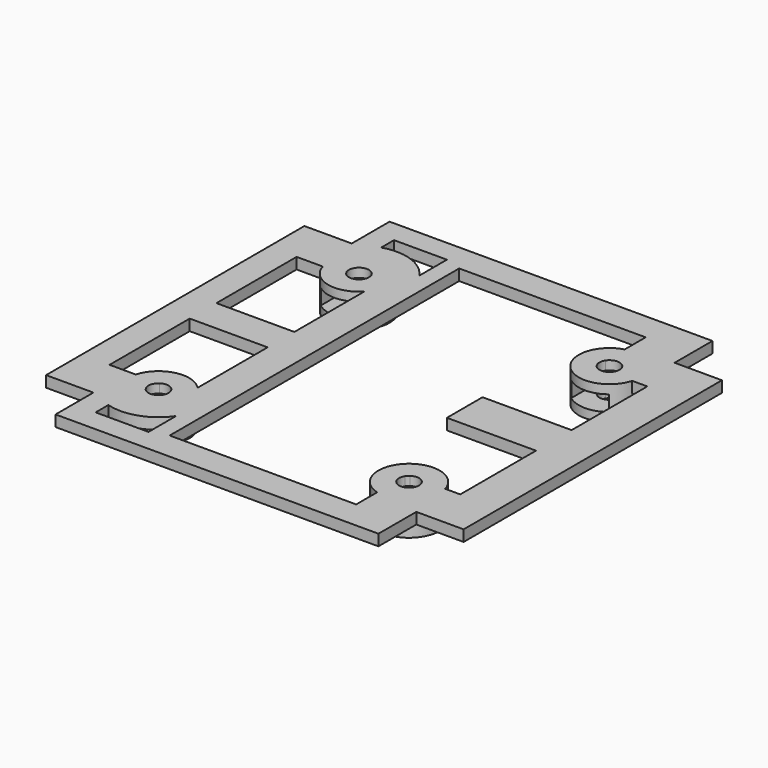
from build123d import *

# Parameters (mm, degrees)
F2_DEPTH       = 2
F3_W           = 13.9999988079
F3_H           = 18
F4_DEPTH       = 2.001
F6_DEPTH       = 6
F7_R           = 1.8
F8_DEPTH       = 6.001
F10_R          = 3.4
F11_DEPTH      = 1.4
F11_DEPTH_BACK = 1.4
F13_W          = 6.8
F13_H          = 2.8
F14_DEPTH      = 8.8
F16_W          = 6.8
F16_H          = 2.8
F17_DEPTH      = 10.3
F18_W          = 8
F18_H          = 2
F19_DEPTH      = 16
F21_DEPTH      = 2.001


# Not quite as in the source:
# - after a boolean that leaves OpenCascade's solid faulty, fix() repairs it
# - a feature names something its author has since deleted; it is built from what else it names


with BuildPart() as f2:
    # F1 (on Top) → F2 (new body)
    with BuildSketch(Plane.XY):
        Polygon((29, 29), (29, 37.5), (-29, 37.5), (-29, 29), (-37.5, 29), (-37.5, -29), (-29, -29), (-29, -37.5), (29, -37.5), (29, -29), (37.5, -29), (37.5, 29), align=None)
    extrude(amount=F2_DEPTH)

    # F3 (on face) → F4 (cut, through all)
    with BuildSketch(Plane.XY.offset(2)):
        with Locations((-25.499999404, 12)):
            Rectangle(F3_W, F3_H)
        with Locations((-25.499999404, -12)):
            Rectangle(F3_W, F3_H)
        Polygon((-12.5, -32.5), (21, -32.5), (21, -21), (30.5, -21), (30.5, 21), (21, 21), (21, 32.5), (-12.5, 32.5), align=None)
    extrude(amount=-F4_DEPTH, mode=Mode.SUBTRACT)

    # F5 (on face) → F6 (join)
    with BuildSketch(Plane.XY.offset(2)):
        with BuildLine():
            ThreePointArc((-23.4949874371, 21), (-23.3511822993, 24.0860292221), (-20.7, 22.5))
            ThreePointArc((-20.7, 22.5), (-20.9139707779, 21.6488177007), (-21.5050125629, 21))
            Line((-21.5050125629, 21), (-18.5, 21))
            Line((-18.5, 21), (-18.5, 18.7250827824))
            ThreePointArc((-18.5, 18.7250827824), (-17.3887379249, 20.4689903988), (-17, 22.5))
            ThreePointArc((-17, 22.5), (-23.2572105316, 27.9476262914), (-27.7915026221, 21))
            Line((-27.7915026221, 21), (-23.4949874371, 21))
        make_face()
        with BuildLine():
            ThreePointArc((-21.5050125629, 21), (-22.5, 20.7), (-23.4949874371, 21))
            Line((-23.4949874371, 21), (-27.7915026221, 21))
            ThreePointArc((-27.7915026221, 21), (-23.8079781506, 17.1577913596), (-18.5, 18.7250827824))
            Line((-18.5, 18.7250827824), (-18.5, 21))
            Line((-18.5, 21), (-21.5050125629, 21))
        make_face()
        with BuildLine():
            ThreePointArc((-21.5050125629, -21), (-20.9139707779, -21.6488177007), (-20.7, -22.5))
            ThreePointArc((-20.7, -22.5), (-23.3511822993, -24.0860292221), (-23.4949874371, -21))
            Line((-23.4949874371, -21), (-27.7915026221, -21))
            ThreePointArc((-27.7915026221, -21), (-23.2572105316, -27.9476262914), (-17, -22.5))
            ThreePointArc((-17, -22.5), (-17.3887379249, -20.4689903988), (-18.5, -18.7250827824))
            Line((-18.5, -18.7250827824), (-18.5, -21))
            Line((-18.5, -21), (-21.5050125629, -21))
        make_face()
        with BuildLine():
            ThreePointArc((-23.4949874371, -21), (-22.5, -20.7), (-21.5050125629, -21))
            Line((-21.5050125629, -21), (-18.5, -21))
            Line((-18.5, -21), (-18.5, -18.7250827824))
            ThreePointArc((-18.5, -18.7250827824), (-23.8079781506, -17.1577913596), (-27.7915026221, -21))
            Line((-27.7915026221, -21), (-23.4949874371, -21))
        make_face()
        with BuildLine():
            ThreePointArc((21, 23.4949874371), (23.0196152423, 24.223368794), (24.3, 22.5))
            ThreePointArc((24.3, 22.5), (24.0860292221, 21.6488177007), (23.4949874371, 21))
            Line((23.4949874371, 21), (27.7915026221, 21))
            ThreePointArc((27.7915026221, 21), (27.9476262914, 21.7427894684), (28, 22.5))
            ThreePointArc((28, 22.5), (25.8166247904, 26.8874821937), (21, 27.7915026221))
            Line((21, 27.7915026221), (21, 23.4949874371))
        make_face()
        with BuildLine():
            ThreePointArc((21, 21.5050125629), (20.7, 22.5), (21, 23.4949874371))
            Line((21, 23.4949874371), (21, 27.7915026221))
            ThreePointArc((21, 27.7915026221), (18.6109127035, 18.6109127035), (27.7915026221, 21))
            Line((27.7915026221, 21), (23.4949874371, 21))
            ThreePointArc((23.4949874371, 21), (22.5, 20.7), (21.5050125629, 21))
            Line((21.5050125629, 21), (21, 21))
            Line((21, 21), (21, 21.5050125629))
        make_face()
        with BuildLine():
            ThreePointArc((21.5050125629, 21), (21.2272077939, 21.2272077939), (21, 21.5050125629))
            Line((21, 21.5050125629), (21, 21))
            Line((21, 21), (21.5050125629, 21))
        make_face()
        with BuildLine():
            Line((23.4949874371, -21), (27.7915026221, -21))
            ThreePointArc((27.7915026221, -21), (18.6109127035, -18.6109127035), (21, -27.7915026221))
            Line((21, -27.7915026221), (21, -23.4949874371))
            ThreePointArc((21, -23.4949874371), (20.7, -22.5), (21, -21.5050125629))
            Line((21, -21.5050125629), (21, -21))
            Line((21, -21), (21.5050125629, -21))
            ThreePointArc((21.5050125629, -21), (22.5, -20.7), (23.4949874371, -21))
        make_face()
        with BuildLine():
            ThreePointArc((28, -22.5), (27.9476262914, -21.7427894684), (27.7915026221, -21))
            Line((27.7915026221, -21), (23.4949874371, -21))
            ThreePointArc((23.4949874371, -21), (24.0860292221, -21.6488177007), (24.3, -22.5))
            ThreePointArc((24.3, -22.5), (23.0196152423, -24.223368794), (21, -23.4949874371))
            Line((21, -23.4949874371), (21, -27.7915026221))
            ThreePointArc((21, -27.7915026221), (25.8166247904, -26.8874821937), (28, -22.5))
        make_face()
        with BuildLine():
            ThreePointArc((21, -21.5050125629), (21.2272077939, -21.2272077939), (21.5050125629, -21))
            Line((21.5050125629, -21), (21, -21))
            Line((21, -21), (21, -21.5050125629))
        make_face()
    extrude(amount=-F6_DEPTH)

    # F7 (on face) → F8 (cut, through all)
    with BuildSketch(Plane(origin=(0, 0, -4), x_dir=(1, 0, 0), z_dir=(0, 0, -1))):
        with Locations((-22.5, -22.5)):
            Circle(F7_R)
        with Locations((-22.5, 22.5)):
            Circle(F7_R)
        with Locations((22.5, -22.5)):
            Circle(F7_R)
        with Locations((22.5, 22.5)):
            Circle(F7_R)
    extrude(amount=-F8_DEPTH, mode=Mode.SUBTRACT)

    add(f2.part.fix(), mode=Mode.REPLACE)

    # F10 (on offset) → F11 (cut, two sides)
    with BuildSketch(Plane.XY.offset(-1)) as f11_sk:
        with Locations((22.5, -22.5)):
            Circle(F10_R)
        with Locations((22.5, 22.5)):
            Circle(F10_R)
        with Locations((-22.5, -22.5)):
            Circle(F10_R)
        with Locations((-22.5, 22.5)):
            Circle(F10_R)
    extrude(amount=-F11_DEPTH, mode=Mode.SUBTRACT)
    extrude(f11_sk.sketch, amount=F11_DEPTH_BACK, mode=Mode.SUBTRACT)

    # F13 (on offset) → F14 (cut)
    with BuildSketch(Plane.XZ.offset(22.5)):
        with Locations((22.5, -1)):
            Rectangle(F13_W, F13_H)
        with Locations((-22.5, -1)):
            Rectangle(F13_W, F13_H)
    extrude(amount=-F14_DEPTH, mode=Mode.SUBTRACT)

    # F16 (on offset) → F17 (cut)
    with BuildSketch(Plane.XZ.offset(-22.5)):
        with Locations((22.5, -1)):
            Rectangle(F16_W, F16_H)
        with Locations((-22.5, -1)):
            Rectangle(F16_W, F16_H)
    extrude(amount=F17_DEPTH, mode=Mode.SUBTRACT)

    # F18 (on face) → F19 (join)
    with BuildSketch(Plane(origin=(30.5, 0, 0), x_dir=(0, -1, 0), z_dir=(-1, 0, 0))):
        with Locations((0, 1)):
            Rectangle(F18_W, F18_H)
    extrude(amount=F19_DEPTH)

    # F20 (on face) → F21 (cut, through all)
    with BuildSketch(Plane(origin=(0, 0, 0), x_dir=(1, 0, 0), z_dir=(0, 0, -1))):
        with BuildLine():
            ThreePointArc((-25, 30.6240384046), (-19.7091840098, 30.5287823553), (-15.4999997467, 27.3218250127))
            Line((-15.4999997467, 27.3218250127), (-15.4999997467, 33.5))
            Line((-15.4999997467, 33.5), (-25, 33.5))
            Line((-25, 33.5), (-25, 30.6240384046))
        make_face()
        with BuildLine():
            Line((-25, -33.5), (-15.4999997467, -33.5))
            Line((-15.4999997467, -33.5), (-15.4999997467, -27.3218250127))
            ThreePointArc((-15.4999997467, -27.3218250127), (-19.7091840098, -30.5287823553), (-25, -30.6240384046))
            Line((-25, -30.6240384046), (-25, -33.5))
        make_face()
    extrude(amount=-F21_DEPTH, mode=Mode.SUBTRACT)


solid = f2.part
